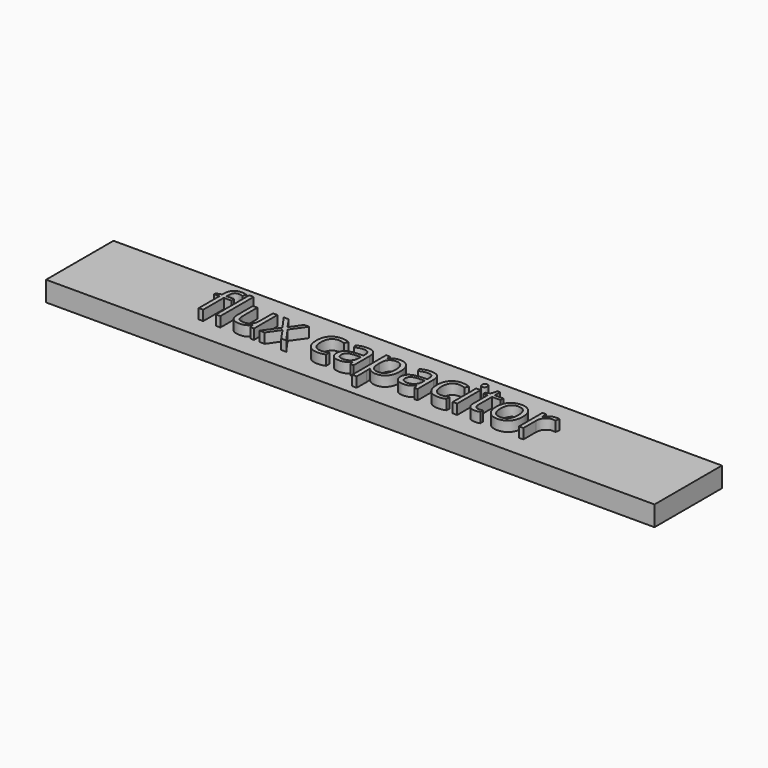
from build123d import *

# Parameters (mm, degrees)
F0_W         = 77.0312733948
F0_H         = 10.6679997407
F0_W_2       = 0.5617585472
F0_H_2       = 3.7071734571
F0_H_3       = 5.2636451158
F1_DEPTH     = 2.54
F0_TEXT_SIZE = 6.9272730293
F2_DEPTH     = 3.81


# Not quite as in the source:
# - Text() gives the source's letters only with a copy of the font that has no kerning and outlines rounded to 1/6400 em; it was checked with that copy


with BuildPart() as f1:
    # F0 (on Top) → F1 (new body)
    with BuildSketch(Plane.XY):
        with Locations((-2.8401818126, -2.4245453533)):
            Rectangle(F0_W, F0_H)
        with BuildLine():
            Line((-20.3521107255, -1.280463124), (-19.7838578598, -1.280463124))
            Line((-19.7838578598, -1.280463124), (-19.7838578598, -3.6855257288))
            add(Edge.make_bspline(
                [(-19.7838578598, -3.6855257288), (-19.7838578598, -4.139045635), (-19.5776632485, -4.3620172356)],
                knots=[0, 0, 0, 1, 1, 1], degree=2))
            add(Edge.make_bspline(
                [(-19.5776632485, -4.3620172356), (-19.3714686373, -4.5849888362), (-18.9320197545, -4.5849888362)],
                knots=[0, 0, 0, 1, 1, 1], degree=2))
            add(Edge.make_bspline(
                [(-18.9320197545, -4.5849888362), (-18.3496958655, -4.5849888362), (-18.0812640356, -4.2673084247)],
                knots=[0, 0, 0, 1, 1, 1], degree=2))
            add(Edge.make_bspline(
                [(-18.0812640356, -4.2673084247), (-17.8128322057, -3.9496280131), (-17.8128322057, -3.2287586635)],
                knots=[0, 0, 0, 1, 1, 1], degree=2))
            Line((-17.8128322057, -3.2287586635), (-17.8128322057, -1.280463124))
            Line((-17.8128322057, -1.280463124), (-17.2510736585, -1.280463124))
            Line((-17.2510736585, -1.280463124), (-17.2510736585, -4.9876365811))
            Line((-17.2510736585, -4.9876365811), (-17.7143350423, -4.9876365811))
            Line((-17.7143350423, -4.9876365811), (-17.7955140231, -4.4908212185))
            Line((-17.7955140231, -4.4908212185), (-17.8258208426, -4.4908212185))
            add(Edge.make_bspline(
                [(-17.8258208426, -4.4908212185), (-17.9979202819, -4.7646649804), (-18.3042356362, -4.9102459527)],
                knots=[0, 0, 0, 1, 1, 1], degree=2))
            add(Edge.make_bspline(
                [(-18.3042356362, -4.9102459527), (-18.6105509905, -5.0558269249), (-19.0034572576, -5.0558269249)],
                knots=[0, 0, 0, 1, 1, 1], degree=2))
            add(Edge.make_bspline(
                [(-19.0034572576, -5.0558269249), (-19.6799487644, -5.0558269249), (-20.0160297449, -4.7343581609)],
                knots=[0, 0, 0, 1, 1, 1], degree=2))
            add(Edge.make_bspline(
                [(-20.0160297449, -4.7343581609), (-20.3521107255, -4.4128893969), (-20.3521107255, -3.7060910707)],
                knots=[0, 0, 0, 1, 1, 1], degree=2))
            Line((-20.3521107255, -3.7060910707), (-20.3521107255, -1.280463124))
        make_face(mode=Mode.SUBTRACT)
        Polygon((-16.5237099904, -4.9876365811), (-15.1674798176, -3.0902132029), (-16.4566020329, -1.280463124), (-15.8169116641, -1.280463124), (-14.8395167352, -2.700554095), (-13.8653689654, -1.280463124), (-13.2321729151, -1.280463124), (-14.5212951304, -3.0902132029), (-13.1650649576, -4.9876365811), (-13.8004257808, -4.9876365811), (-14.8395167352, -3.4852842428), (-15.8883491672, -4.9876365811), align=None, mode=Mode.SUBTRACT)
        with BuildLine():
            add(Edge.make_bspline(
                [(-8.2131471281, -4.8620797574), (-8.584405667, -5.0558269249), (-9.1494113735, -5.0558269249)],
                knots=[0, 0, 0, 1, 1, 1], degree=2))
            add(Edge.make_bspline(
                [(-9.1494113735, -5.0558269249), (-9.9547068631, -5.0558269249), (-10.3963205187, -4.5600939488)],
                knots=[0, 0, 0, 1, 1, 1], degree=2))
            add(Edge.make_bspline(
                [(-10.3963205187, -4.5600939488), (-10.8379341744, -4.0643609726), (-10.8379341744, -3.1573211604)],
                knots=[0, 0, 0, 1, 1, 1], degree=2))
            add(Edge.make_bspline(
                [(-10.8379341744, -3.1573211604), (-10.8379341744, -2.2275512335), (-10.3892850071, -1.7199120068)],
                knots=[0, 0, 0, 1, 1, 1], degree=2))
            add(Edge.make_bspline(
                [(-10.3892850071, -1.7199120068), (-9.9406358398, -1.2122727801), (-9.1126102355, -1.2122727801)],
                knots=[0, 0, 0, 1, 1, 1], degree=2))
            add(Edge.make_bspline(
                [(-9.1126102355, -1.2122727801), (-8.845260792, -1.2122727801), (-8.5779113486, -1.2701804531)],
                knots=[0, 0, 0, 1, 1, 1], degree=2))
            add(Edge.make_bspline(
                [(-8.5779113486, -1.2701804531), (-8.3105619051, -1.3280881261), (-8.1590278076, -1.4060199477)],
                knots=[0, 0, 0, 1, 1, 1], degree=2))
            Line((-8.1590278076, -1.4060199477), (-8.3311272469, -1.8822699684))
            add(Edge.make_bspline(
                [(-8.3311272469, -1.8822699684), (-8.5172977096, -1.8075853061), (-8.737022151, -1.7588779176)],
                knots=[0, 0, 0, 1, 1, 1], degree=2))
            add(Edge.make_bspline(
                [(-8.737022151, -1.7588779176), (-8.9567465924, -1.7101705291), (-9.1255988724, -1.7101705291)],
                knots=[0, 0, 0, 1, 1, 1], degree=2))
            add(Edge.make_bspline(
                [(-9.1255988724, -1.7101705291), (-10.2556102853, -1.7101705291), (-10.2556102853, -3.1508268419)],
                knots=[0, 0, 0, 1, 1, 1], degree=2))
            add(Edge.make_bspline(
                [(-10.2556102853, -3.1508268419), (-10.2556102853, -3.8338126671), (-9.9801429438, -4.1991180808)],
                knots=[0, 0, 0, 1, 1, 1], degree=2))
            add(Edge.make_bspline(
                [(-9.9801429438, -4.1991180808), (-9.7046756022, -4.5644234944), (-9.1634823968, -4.5644234944)],
                knots=[0, 0, 0, 1, 1, 1], degree=2))
            add(Edge.make_bspline(
                [(-9.1634823968, -4.5644234944), (-8.700221013, -4.5644234944), (-8.2131471281, -4.3652643948)],
                knots=[0, 0, 0, 1, 1, 1], degree=2))
            Line((-8.2131471281, -4.3652643948), (-8.2131471281, -4.8620797574))
        make_face(mode=Mode.SUBTRACT)
        with BuildLine():
            Line((-4.6369424268, -4.9876365811), (-5.0536611949, -4.9876365811))
            Line((-5.0536611949, -4.9876365811), (-5.1651469952, -4.4594320126))
            Line((-5.1651469952, -4.4594320126), (-5.1922066555, -4.4594320126))
            add(Edge.make_bspline(
                [(-5.1922066555, -4.4594320126), (-5.4692975767, -4.8079604369), (-5.7447649182, -4.9318936809)],
                knots=[0, 0, 0, 1, 1, 1], degree=2))
            add(Edge.make_bspline(
                [(-5.7447649182, -4.9318936809), (-6.0202322598, -5.0558269249), (-6.4337038687, -5.0558269249)],
                knots=[0, 0, 0, 1, 1, 1], degree=2))
            add(Edge.make_bspline(
                [(-6.4337038687, -5.0558269249), (-6.9846385518, -5.0558269249), (-7.2974482246, -4.7711592989)],
                knots=[0, 0, 0, 1, 1, 1], degree=2))
            add(Edge.make_bspline(
                [(-7.2974482246, -4.7711592989), (-7.6102578973, -4.4864916729), (-7.6102578973, -3.96261665)],
                knots=[0, 0, 0, 1, 1, 1], degree=2))
            add(Edge.make_bspline(
                [(-7.6102578973, -3.96261665), (-7.6102578973, -2.840181942), (-5.8145788417, -2.7860626215)],
                knots=[0, 0, 0, 1, 1, 1], degree=2))
            Line((-5.8145788417, -2.7860626215), (-5.1857123371, -2.7654972796))
            Line((-5.1857123371, -2.7654972796), (-5.1857123371, -2.5349489741))
            add(Edge.make_bspline(
                [(-5.1857123371, -2.5349489741), (-5.1857123371, -2.0987472506), (-5.3729651861, -1.8909290597)],
                knots=[0, 0, 0, 1, 1, 1], degree=2))
            add(Edge.make_bspline(
                [(-5.3729651861, -1.8909290597), (-5.5602180352, -1.6831108688), (-5.9736896441, -1.6831108688)],
                knots=[0, 0, 0, 1, 1, 1], degree=2))
            add(Edge.make_bspline(
                [(-5.9736896441, -1.6831108688), (-6.436951028, -1.6831108688), (-7.0214396898, -1.9666961085)],
                knots=[0, 0, 0, 1, 1, 1], degree=2))
            Line((-7.0214396898, -1.9666961085), (-7.1946215155, -1.5369887034))
            add(Edge.make_bspline(
                [(-7.1946215155, -1.5369887034), (-6.9207777536, -1.3887017651), (-6.5944382507, -1.304275625)],
                knots=[0, 0, 0, 1, 1, 1], degree=2))
            add(Edge.make_bspline(
                [(-6.5944382507, -1.304275625), (-6.2680987479, -1.219849485), (-5.939053279, -1.219849485)],
                knots=[0, 0, 0, 1, 1, 1], degree=2))
            add(Edge.make_bspline(
                [(-5.939053279, -1.219849485), (-5.2766327956, -1.219849485), (-4.9567876112, -1.5137173955)],
                knots=[0, 0, 0, 1, 1, 1], degree=2))
            add(Edge.make_bspline(
                [(-4.9567876112, -1.5137173955), (-4.6369424268, -1.8075853061), (-4.6369424268, -2.4570171526)],
                knots=[0, 0, 0, 1, 1, 1], degree=2))
            Line((-4.6369424268, -2.4570171526), (-4.6369424268, -4.9876365811))
        make_face(mode=Mode.SUBTRACT)
        with BuildLine():
            add(Edge.make_bspline(
                [(-0.6239948086, -4.5498112779), (-1.0315132923, -5.0558269249), (-1.7556298012, -5.0558269249)],
                knots=[0, 0, 0, 1, 1, 1], degree=2))
            add(Edge.make_bspline(
                [(-1.7556298012, -5.0558269249), (-2.1182292488, -5.0558269249), (-2.4175090914, -4.9221522032)],
                knots=[0, 0, 0, 1, 1, 1], degree=2))
            add(Edge.make_bspline(
                [(-2.4175090914, -4.9221522032), (-2.716788934, -4.7884774815), (-2.9191951928, -4.5103041739)],
                knots=[0, 0, 0, 1, 1, 1], degree=2))
            Line((-2.9191951928, -4.5103041739), (-2.9603258764, -4.5103041739))
            add(Edge.make_bspline(
                [(-2.9603258764, -4.5103041739), (-2.9191951928, -4.8350200971), (-2.9191951928, -5.1261820416)],
                knots=[0, 0, 0, 1, 1, 1], degree=2))
            Line((-2.9191951928, -5.1261820416), (-2.9191951928, -6.6523468809))
            Line((-2.9191951928, -6.6523468809), (-3.48095374, -6.6523468809))
            Line((-3.48095374, -6.6523468809), (-3.48095374, -1.280463124))
            Line((-3.48095374, -1.280463124), (-3.0241866746, -1.280463124))
            Line((-3.0241866746, -1.280463124), (-2.9462548531, -1.7881023507))
            Line((-2.9462548531, -1.7881023507), (-2.9191951928, -1.7881023507))
            add(Edge.make_bspline(
                [(-2.9191951928, -1.7881023507), (-2.7027179106, -1.4828693828), (-2.4153443186, -1.3475710815)],
                knots=[0, 0, 0, 1, 1, 1], degree=2))
            add(Edge.make_bspline(
                [(-2.4153443186, -1.3475710815), (-2.1279707265, -1.2122727801), (-1.7556298012, -1.2122727801)],
                knots=[0, 0, 0, 1, 1, 1], degree=2))
            add(Edge.make_bspline(
                [(-1.7556298012, -1.2122727801), (-1.0185246554, -1.2122727801), (-0.6175004902, -1.7166648476)],
                knots=[0, 0, 0, 1, 1, 1], degree=2))
            add(Edge.make_bspline(
                [(-0.6175004902, -1.7166648476), (-0.216476325, -2.221056915), (-0.216476325, -3.1302615001)],
                knots=[0, 0, 0, 1, 1, 1], degree=2))
            add(Edge.make_bspline(
                [(-0.216476325, -3.1302615001), (-0.216476325, -4.0437956308), (-0.6239948086, -4.5498112779)],
                knots=[0, 0, 0, 1, 1, 1], degree=2))
        make_face(mode=Mode.SUBTRACT)
        with BuildLine():
            Line((3.4603903126, -4.9876365811), (3.0436715444, -4.9876365811))
            Line((3.0436715444, -4.9876365811), (2.9321857441, -4.4594320126))
            Line((2.9321857441, -4.4594320126), (2.9051260838, -4.4594320126))
            add(Edge.make_bspline(
                [(2.9051260838, -4.4594320126), (2.6280351627, -4.8079604369), (2.3525678211, -4.9318936809)],
                knots=[0, 0, 0, 1, 1, 1], degree=2))
            add(Edge.make_bspline(
                [(2.3525678211, -4.9318936809), (2.0771004796, -5.0558269249), (1.6636288706, -5.0558269249)],
                knots=[0, 0, 0, 1, 1, 1], degree=2))
            add(Edge.make_bspline(
                [(1.6636288706, -5.0558269249), (1.1126941875, -5.0558269249), (0.7998845148, -4.7711592989)],
                knots=[0, 0, 0, 1, 1, 1], degree=2))
            add(Edge.make_bspline(
                [(0.7998845148, -4.7711592989), (0.4870748421, -4.4864916729), (0.4870748421, -3.96261665)],
                knots=[0, 0, 0, 1, 1, 1], degree=2))
            add(Edge.make_bspline(
                [(0.4870748421, -3.96261665), (0.4870748421, -2.840181942), (2.2827538976, -2.7860626215)],
                knots=[0, 0, 0, 1, 1, 1], degree=2))
            Line((2.2827538976, -2.7860626215), (2.9116204023, -2.7654972796))
            Line((2.9116204023, -2.7654972796), (2.9116204023, -2.5349489741))
            add(Edge.make_bspline(
                [(2.9116204023, -2.5349489741), (2.9116204023, -2.0987472506), (2.7243675532, -1.8909290597)],
                knots=[0, 0, 0, 1, 1, 1], degree=2))
            add(Edge.make_bspline(
                [(2.7243675532, -1.8909290597), (2.5371147042, -1.6831108688), (2.1236430952, -1.6831108688)],
                knots=[0, 0, 0, 1, 1, 1], degree=2))
            add(Edge.make_bspline(
                [(2.1236430952, -1.6831108688), (1.6603817114, -1.6831108688), (1.0758930495, -1.9666961085)],
                knots=[0, 0, 0, 1, 1, 1], degree=2))
            Line((1.0758930495, -1.9666961085), (0.9027112238, -1.5369887034))
            add(Edge.make_bspline(
                [(0.9027112238, -1.5369887034), (1.1765549858, -1.3887017651), (1.5028944886, -1.304275625)],
                knots=[0, 0, 0, 1, 1, 1], degree=2))
            add(Edge.make_bspline(
                [(1.5028944886, -1.304275625), (1.8292339915, -1.219849485), (2.1582794604, -1.219849485)],
                knots=[0, 0, 0, 1, 1, 1], degree=2))
            add(Edge.make_bspline(
                [(2.1582794604, -1.219849485), (2.8206999438, -1.219849485), (3.1405451282, -1.5137173955)],
                knots=[0, 0, 0, 1, 1, 1], degree=2))
            add(Edge.make_bspline(
                [(3.1405451282, -1.5137173955), (3.4603903126, -1.8075853061), (3.4603903126, -2.4570171526)],
                knots=[0, 0, 0, 1, 1, 1], degree=2))
            Line((3.4603903126, -2.4570171526), (3.4603903126, -4.9876365811))
        make_face(mode=Mode.SUBTRACT)
        with BuildLine():
            add(Edge.make_bspline(
                [(7.0344302411, -4.8620797574), (6.6631717022, -5.0558269249), (6.0981659958, -5.0558269249)],
                knots=[0, 0, 0, 1, 1, 1], degree=2))
            add(Edge.make_bspline(
                [(6.0981659958, -5.0558269249), (5.2928705061, -5.0558269249), (4.8512568505, -4.5600939488)],
                knots=[0, 0, 0, 1, 1, 1], degree=2))
            add(Edge.make_bspline(
                [(4.8512568505, -4.5600939488), (4.4096431949, -4.0643609726), (4.4096431949, -3.1573211604)],
                knots=[0, 0, 0, 1, 1, 1], degree=2))
            add(Edge.make_bspline(
                [(4.4096431949, -3.1573211604), (4.4096431949, -2.2275512335), (4.8582923622, -1.7199120068)],
                knots=[0, 0, 0, 1, 1, 1], degree=2))
            add(Edge.make_bspline(
                [(4.8582923622, -1.7199120068), (5.3069415294, -1.2122727801), (6.1349671337, -1.2122727801)],
                knots=[0, 0, 0, 1, 1, 1], degree=2))
            add(Edge.make_bspline(
                [(6.1349671337, -1.2122727801), (6.4023165772, -1.2122727801), (6.6696660207, -1.2701804531)],
                knots=[0, 0, 0, 1, 1, 1], degree=2))
            add(Edge.make_bspline(
                [(6.6696660207, -1.2701804531), (6.9370154641, -1.3280881261), (7.0885495617, -1.4060199477)],
                knots=[0, 0, 0, 1, 1, 1], degree=2))
            Line((7.0885495617, -1.4060199477), (6.9164501223, -1.8822699684))
            add(Edge.make_bspline(
                [(6.9164501223, -1.8822699684), (6.7302796597, -1.8075853061), (6.5105552183, -1.7588779176)],
                knots=[0, 0, 0, 1, 1, 1], degree=2))
            add(Edge.make_bspline(
                [(6.5105552183, -1.7588779176), (6.2908307769, -1.7101705291), (6.1219784968, -1.7101705291)],
                knots=[0, 0, 0, 1, 1, 1], degree=2))
            add(Edge.make_bspline(
                [(6.1219784968, -1.7101705291), (4.9919670839, -1.7101705291), (4.9919670839, -3.1508268419)],
                knots=[0, 0, 0, 1, 1, 1], degree=2))
            add(Edge.make_bspline(
                [(4.9919670839, -3.1508268419), (4.9919670839, -3.8338126671), (5.2674344255, -4.1991180808)],
                knots=[0, 0, 0, 1, 1, 1], degree=2))
            add(Edge.make_bspline(
                [(5.2674344255, -4.1991180808), (5.542901767, -4.5644234944), (6.0840949724, -4.5644234944)],
                knots=[0, 0, 0, 1, 1, 1], degree=2))
            add(Edge.make_bspline(
                [(6.0840949724, -4.5644234944), (6.5473563562, -4.5644234944), (7.0344302411, -4.3652643948)],
                knots=[0, 0, 0, 1, 1, 1], degree=2))
            Line((7.0344302411, -4.3652643948), (7.0344302411, -4.8620797574))
        make_face(mode=Mode.SUBTRACT)
        with Locations((8.1952896667, -3.1340498525)):
            Rectangle(F0_W_2, F0_H_2, mode=Mode.SUBTRACT)
        with BuildLine():
            add(Edge.make_bspline(
                [(14.8530484797, -1.7301946777), (15.3114391247, -2.2481165753), (15.3114391247, -3.1302615001)],
                knots=[0, 0, 0, 1, 1, 1], degree=2))
            add(Edge.make_bspline(
                [(15.3114391247, -3.1302615001), (15.3114391247, -4.0373013124), (14.8552132525, -4.5465641187)],
                knots=[0, 0, 0, 1, 1, 1], degree=2))
            add(Edge.make_bspline(
                [(14.8552132525, -4.5465641187), (14.3989873803, -5.0558269249), (13.5936918907, -5.0558269249)],
                knots=[0, 0, 0, 1, 1, 1], degree=2))
            add(Edge.make_bspline(
                [(13.5936918907, -5.0558269249), (13.0957941417, -5.0558269249), (12.7104645795, -4.8220314602)],
                knots=[0, 0, 0, 1, 1, 1], degree=2))
            add(Edge.make_bspline(
                [(12.7104645795, -4.8220314602), (12.3251350172, -4.5882359955), (12.1151520535, -4.1520342719)],
                knots=[0, 0, 0, 1, 1, 1], degree=2))
            add(Edge.make_bspline(
                [(12.1151520535, -4.1520342719), (11.9051690898, -3.7158325483), (11.9051690898, -3.1302615001)],
                knots=[0, 0, 0, 1, 1, 1], degree=2))
            add(Edge.make_bspline(
                [(11.9051690898, -3.1302615001), (11.9051690898, -2.2243040742), (12.3586889959, -1.7182884272)],
                knots=[0, 0, 0, 1, 1, 1], degree=2))
            add(Edge.make_bspline(
                [(12.3586889959, -1.7182884272), (12.8122089021, -1.2122727801), (13.6175043917, -1.2122727801)],
                knots=[0, 0, 0, 1, 1, 1], degree=2))
            add(Edge.make_bspline(
                [(13.6175043917, -1.2122727801), (14.3946578347, -1.2122727801), (14.8530484797, -1.7301946777)],
                knots=[0, 0, 0, 1, 1, 1], degree=2))
        make_face(mode=Mode.SUBTRACT)
        with BuildLine():
            add(Edge.make_bspline(
                [(10.427711639, -4.4123482037), (10.5868224414, -4.5914831547), (10.8639133626, -4.5914831547)],
                knots=[0, 0, 0, 1, 1, 1], degree=2))
            add(Edge.make_bspline(
                [(10.8639133626, -4.5914831547), (11.0132826873, -4.5914831547), (11.1518281479, -4.5698354265)],
                knots=[0, 0, 0, 1, 1, 1], degree=2))
            add(Edge.make_bspline(
                [(11.1518281479, -4.5698354265), (11.2903736085, -4.5481876983), (11.3715525893, -4.5243751972)],
                knots=[0, 0, 0, 1, 1, 1], degree=2))
            Line((11.3715525893, -4.5243751972), (11.3715525893, -4.9540826023))
            add(Edge.make_bspline(
                [(11.3715525893, -4.9540826023), (11.2806321308, -4.9973780588), (11.1031207594, -5.0266024919)],
                knots=[0, 0, 0, 1, 1, 1], degree=2))
            add(Edge.make_bspline(
                [(11.1031207594, -5.0266024919), (10.925609388, -5.0558269249), (10.7827343818, -5.0558269249)],
                knots=[0, 0, 0, 1, 1, 1], degree=2))
            add(Edge.make_bspline(
                [(10.7827343818, -5.0558269249), (9.7079246758, -5.0558269249), (9.7079246758, -3.9225683528)],
                knots=[0, 0, 0, 1, 1, 1], degree=2))
            Line((9.7079246758, -3.9225683528), (9.7079246758, -1.7166648476))
            Line((9.7079246758, -1.7166648476), (9.1764729481, -1.7166648476))
            Line((9.1764729481, -1.7166648476), (9.1764729481, -1.4460682449))
            Line((9.1764729481, -1.4460682449), (9.7079246758, -1.2122727801))
            Line((9.7079246758, -1.2122727801), (9.9438849134, -0.4210483138))
            Line((9.9438849134, -0.4210483138), (10.2686008367, -0.4210483138))
            Line((10.2686008367, -0.4210483138), (10.2686008367, -1.280463124))
            Line((10.2686008367, -1.280463124), (11.344492929, -1.280463124))
            Line((11.344492929, -1.280463124), (11.344492929, -1.7166648476))
            Line((11.344492929, -1.7166648476), (10.2686008367, -1.7166648476))
            Line((10.2686008367, -1.7166648476), (10.2686008367, -3.8987558518))
            add(Edge.make_bspline(
                [(10.2686008367, -3.8987558518), (10.2686008367, -4.2332132527), (10.427711639, -4.4123482037)],
                knots=[0, 0, 0, 1, 1, 1], degree=2))
        make_face(mode=Mode.SUBTRACT)
        with BuildLine():
            add(Edge.make_bspline(
                [(17.3484903498, -1.4087259137), (17.6396522943, -1.2122727801), (17.9881807186, -1.2122727801)],
                knots=[0, 0, 0, 1, 1, 1], degree=2))
            add(Edge.make_bspline(
                [(17.9881807186, -1.2122727801), (18.2349648203, -1.2122727801), (18.4308767607, -1.2534034637)],
                knots=[0, 0, 0, 1, 1, 1], degree=2))
            Line((18.4308767607, -1.2534034637), (18.3529449391, -1.7740313273))
            add(Edge.make_bspline(
                [(18.3529449391, -1.7740313273), (18.12347902, -1.723159166), (17.947050035, -1.723159166)],
                knots=[0, 0, 0, 1, 1, 1], degree=2))
            add(Edge.make_bspline(
                [(17.947050035, -1.723159166), (17.4967772881, -1.723159166), (17.1774732969, -2.0884645797)],
                knots=[0, 0, 0, 1, 1, 1], degree=2))
            add(Edge.make_bspline(
                [(17.1774732969, -2.0884645797), (16.8581693057, -2.4537699933), (16.8581693057, -2.998210358)],
                knots=[0, 0, 0, 1, 1, 1], degree=2))
            Line((16.8581693057, -2.998210358), (16.8581693057, -4.9876365811))
            Line((16.8581693057, -4.9876365811), (16.2964107585, -4.9876365811))
            Line((16.2964107585, -4.9876365811), (16.2964107585, -1.280463124))
            Line((16.2964107585, -1.280463124), (16.7596721423, -1.280463124))
            Line((16.7596721423, -1.280463124), (16.824615327, -1.9666961085))
            Line((16.824615327, -1.9666961085), (16.8516749873, -1.9666961085))
            add(Edge.make_bspline(
                [(16.8516749873, -1.9666961085), (17.0573284053, -1.6051790472), (17.3484903498, -1.4087259137)],
                knots=[0, 0, 0, 1, 1, 1], degree=2))
        make_face(mode=Mode.SUBTRACT)
        with BuildLine():
            Line((-22.7409375342, -1.280463124), (-22.7409375342, -1.7166648476))
            Line((-22.7409375342, -1.7166648476), (-23.6847784844, -1.7166648476))
            Line((-23.6847784844, -1.7166648476), (-23.6847784844, -4.9876365811))
            Line((-23.6847784844, -4.9876365811), (-24.2465370316, -4.9876365811))
            Line((-24.2465370316, -4.9876365811), (-24.2465370316, -1.7166648476))
            Line((-24.2465370316, -1.7166648476), (-24.908957515, -1.7166648476))
            Line((-24.908957515, -1.7166648476), (-24.908957515, -1.4633864274))
            Line((-24.908957515, -1.4633864274), (-24.2465370316, -1.2598977822))
            Line((-24.2465370316, -1.2598977822), (-24.2465370316, -1.0542443641))
            add(Edge.make_bspline(
                [(-24.2465370316, -1.0542443641), (-24.2465370316, 0.3128096727), (-23.0526648205, 0.3128096727)],
                knots=[0, 0, 0, 1, 1, 1], degree=2))
            add(Edge.make_bspline(
                [(-23.0526648205, 0.3128096727), (-22.7582557167, 0.3128096727), (-22.3621022904, 0.1948295539)],
                knots=[0, 0, 0, 1, 1, 1], degree=2))
            Line((-22.3621022904, 0.1948295539), (-22.5082244558, -0.255443193))
            add(Edge.make_bspline(
                [(-22.5082244558, -0.255443193), (-22.8329403791, -0.1504517111), (-23.0624062982, -0.1504517111)],
                knots=[0, 0, 0, 1, 1, 1], degree=2))
            add(Edge.make_bspline(
                [(-23.0624062982, -0.1504517111), (-23.380627903, -0.1504517111), (-23.5327031937, -0.3620582544)],
                knots=[0, 0, 0, 1, 1, 1], degree=2))
            add(Edge.make_bspline(
                [(-23.5327031937, -0.3620582544), (-23.6847784844, -0.5736647977), (-23.6847784844, -1.0401733408)],
                knots=[0, 0, 0, 1, 1, 1], degree=2))
            Line((-23.6847784844, -1.0401733408), (-23.6847784844, -1.280463124))
            Line((-23.6847784844, -1.280463124), (-22.7409375342, -1.280463124))
        make_face(mode=Mode.SUBTRACT)
        with Locations((-21.7835667538, -2.3558140232)):
            Rectangle(F0_W_2, F0_H_3, mode=Mode.SUBTRACT)
        with BuildLine():
            add(Edge.make_bspline(
                [(7.961494202, -0.558511388), (7.866785391, -0.4654261567), (7.866785391, -0.2760085348)],
                knots=[0, 0, 0, 1, 1, 1], degree=2))
            add(Edge.make_bspline(
                [(7.866785391, -0.2760085348), (7.866785391, -0.0833437536), (7.961494202, 0.0064943185)],
                knots=[0, 0, 0, 1, 1, 1], degree=2))
            add(Edge.make_bspline(
                [(7.961494202, 0.0064943185), (8.0562030129, 0.0963323906), (8.1990780192, 0.0963323906)],
                knots=[0, 0, 0, 1, 1, 1], degree=2))
            add(Edge.make_bspline(
                [(8.1990780192, 0.0963323906), (8.3343763205, 0.0963323906), (8.4323322907, 0.0048707388)],
                knots=[0, 0, 0, 1, 1, 1], degree=2))
            add(Edge.make_bspline(
                [(8.4323322907, 0.0048707388), (8.5302882609, -0.0865909129), (8.5302882609, -0.2760085348)],
                knots=[0, 0, 0, 1, 1, 1], degree=2))
            add(Edge.make_bspline(
                [(8.5302882609, -0.2760085348), (8.5302882609, -0.4654261567), (8.4323322907, -0.558511388)],
                knots=[0, 0, 0, 1, 1, 1], degree=2))
            add(Edge.make_bspline(
                [(8.4323322907, -0.558511388), (8.3343763205, -0.6515966193), (8.1990780192, -0.6515966193)],
                knots=[0, 0, 0, 1, 1, 1], degree=2))
            add(Edge.make_bspline(
                [(8.1990780192, -0.6515966193), (8.0562030129, -0.6515966193), (7.961494202, -0.558511388)],
                knots=[0, 0, 0, 1, 1, 1], degree=2))
        make_face(mode=Mode.SUBTRACT)
    extrude(amount=F1_DEPTH)


with BuildPart() as f1b:
    # F0 (on Top) → F1, piece 2 (new body)
    with BuildSketch(Plane.XY):
        with BuildLine():
            add(Edge.make_bspline(
                [(-6.837434, -4.4329135455), (-6.6534283101, -4.5914831547), (-6.3222180684, -4.5914831547)],
                knots=[0, 0, 0, 1, 1, 1], degree=2))
            add(Edge.make_bspline(
                [(-6.3222180684, -4.5914831547), (-5.7972606592, -4.5914831547), (-5.4979808166, -4.3041095626)],
                knots=[0, 0, 0, 1, 1, 1], degree=2))
            add(Edge.make_bspline(
                [(-5.4979808166, -4.3041095626), (-5.198700974, -4.0167359706), (-5.198700974, -3.4993552662)],
                knots=[0, 0, 0, 1, 1, 1], degree=2))
            Line((-5.198700974, -3.4993552662), (-5.198700974, -3.1648978652))
            Line((-5.198700974, -3.1648978652), (-5.7604595212, -3.1876279799))
            add(Edge.make_bspline(
                [(-5.7604595212, -3.1876279799), (-6.4304567095, -3.2114404809), (-6.7259481996, -3.395987364)],
                knots=[0, 0, 0, 1, 1, 1], degree=2))
            add(Edge.make_bspline(
                [(-6.7259481996, -3.395987364), (-7.0214396898, -3.580534247), (-7.0214396898, -3.9691109685)],
                knots=[0, 0, 0, 1, 1, 1], degree=2))
            add(Edge.make_bspline(
                [(-7.0214396898, -3.9691109685), (-7.0214396898, -4.2743439363), (-6.837434, -4.4329135455)],
                knots=[0, 0, 0, 1, 1, 1], degree=2))
        make_face()
    extrude(amount=F1_DEPTH)


with BuildPart() as f1c:
    # F0 (on Top) → F1, piece 3 (new body)
    with BuildSketch(Plane.XY):
        with BuildLine():
            add(Edge.make_bspline(
                [(-1.0710203963, -2.0597813398), (-1.3432405786, -1.6896051873), (-1.836808782, -1.6896051873)],
                knots=[0, 0, 0, 1, 1, 1], degree=2))
            add(Edge.make_bspline(
                [(-1.836808782, -1.6896051873), (-2.4050616477, -1.6896051873), (-2.658881261, -2.0040384396)],
                knots=[0, 0, 0, 1, 1, 1], degree=2))
            add(Edge.make_bspline(
                [(-2.658881261, -2.0040384396), (-2.9127008743, -2.318471692), (-2.9191951928, -3.0057870628)],
                knots=[0, 0, 0, 1, 1, 1], degree=2))
            Line((-2.9191951928, -3.0057870628), (-2.9191951928, -3.1302615001))
            add(Edge.make_bspline(
                [(-2.9191951928, -3.1302615001), (-2.9191951928, -3.9117444887), (-2.658881261, -4.2483666625)],
                knots=[0, 0, 0, 1, 1, 1], degree=2))
            add(Edge.make_bspline(
                [(-2.658881261, -4.2483666625), (-2.3985673292, -4.5849888362), (-1.823820145, -4.5849888362)],
                knots=[0, 0, 0, 1, 1, 1], degree=2))
            add(Edge.make_bspline(
                [(-1.823820145, -4.5849888362), (-1.3432405786, -4.5849888362), (-1.0710203963, -4.1958709215)],
                knots=[0, 0, 0, 1, 1, 1], degree=2))
            add(Edge.make_bspline(
                [(-1.0710203963, -4.1958709215), (-0.798800214, -3.8067530069), (-0.798800214, -3.1237671816)],
                knots=[0, 0, 0, 1, 1, 1], degree=2))
            add(Edge.make_bspline(
                [(-0.798800214, -3.1237671816), (-0.798800214, -2.4299574923), (-1.0710203963, -2.0597813398)],
                knots=[0, 0, 0, 1, 1, 1], degree=2))
        make_face()
    extrude(amount=F1_DEPTH)


with BuildPart() as f1d:
    # F0 (on Top) → F1, piece 4 (new body)
    with BuildSketch(Plane.XY):
        with BuildLine():
            add(Edge.make_bspline(
                [(1.2598987394, -4.4329135455), (1.4439044292, -4.5914831547), (1.7751146709, -4.5914831547)],
                knots=[0, 0, 0, 1, 1, 1], degree=2))
            add(Edge.make_bspline(
                [(1.7751146709, -4.5914831547), (2.3000720802, -4.5914831547), (2.5993519228, -4.3041095626)],
                knots=[0, 0, 0, 1, 1, 1], degree=2))
            add(Edge.make_bspline(
                [(2.5993519228, -4.3041095626), (2.8986317654, -4.0167359706), (2.8986317654, -3.4993552662)],
                knots=[0, 0, 0, 1, 1, 1], degree=2))
            Line((2.8986317654, -3.4993552662), (2.8986317654, -3.1648978652))
            Line((2.8986317654, -3.1648978652), (2.3368732182, -3.1876279799))
            add(Edge.make_bspline(
                [(2.3368732182, -3.1876279799), (1.6668760299, -3.2114404809), (1.3713845397, -3.395987364)],
                knots=[0, 0, 0, 1, 1, 1], degree=2))
            add(Edge.make_bspline(
                [(1.3713845397, -3.395987364), (1.0758930495, -3.580534247), (1.0758930495, -3.9691109685)],
                knots=[0, 0, 0, 1, 1, 1], degree=2))
            add(Edge.make_bspline(
                [(1.0758930495, -3.9691109685), (1.0758930495, -4.2743439363), (1.2598987394, -4.4329135455)],
                knots=[0, 0, 0, 1, 1, 1], degree=2))
        make_face()
    extrude(amount=F1_DEPTH)


with BuildPart() as f1e:
    # F0 (on Top) → F1, piece 5 (new body)
    with BuildSketch(Plane.XY):
        with BuildLine():
            add(Edge.make_bspline(
                [(12.7683722524, -2.0516634417), (12.4874929788, -2.4137216961), (12.4874929788, -3.1302615001)],
                knots=[0, 0, 0, 1, 1, 1], degree=2))
            add(Edge.make_bspline(
                [(12.4874929788, -3.1302615001), (12.4874929788, -3.841389372), (12.7716194117, -4.2131891041)],
                knots=[0, 0, 0, 1, 1, 1], degree=2))
            add(Edge.make_bspline(
                [(12.7716194117, -4.2131891041), (13.0557458445, -4.5849888362), (13.6066805276, -4.5849888362)],
                knots=[0, 0, 0, 1, 1, 1], degree=2))
            add(Edge.make_bspline(
                [(13.6066805276, -4.5849888362), (14.1586975971, -4.5849888362), (14.4444476096, -4.2148126837)],
                knots=[0, 0, 0, 1, 1, 1], degree=2))
            add(Edge.make_bspline(
                [(14.4444476096, -4.2148126837), (14.7301976221, -3.8446365312), (14.7301976221, -3.1302615001)],
                knots=[0, 0, 0, 1, 1, 1], degree=2))
            add(Edge.make_bspline(
                [(14.7301976221, -3.1302615001), (14.7301976221, -2.4234631738), (14.4444476096, -2.0565341806)],
                knots=[0, 0, 0, 1, 1, 1], degree=2))
            add(Edge.make_bspline(
                [(14.4444476096, -2.0565341806), (14.1586975971, -1.6896051873), (13.6001862092, -1.6896051873)],
                knots=[0, 0, 0, 1, 1, 1], degree=2))
            add(Edge.make_bspline(
                [(13.6001862092, -1.6896051873), (13.0492515261, -1.6896051873), (12.7683722524, -2.0516634417)],
                knots=[0, 0, 0, 1, 1, 1], degree=2))
        make_face()
    extrude(amount=F1_DEPTH)


with BuildPart() as f2:
    # F0 (on Top) → F2 (new body)
    with BuildSketch(Plane.XY):
        with Locations((-25.0074546784, -4.9876365811)):
            Text('flux capacitor', F0_TEXT_SIZE, font='Open Sans', text_align=(TextAlign.LEFT, TextAlign.BOTTOM))
    extrude(amount=F2_DEPTH)


solid = Compound([f1.part, f1b.part, f1c.part, f1d.part, f1e.part, f2.part])
